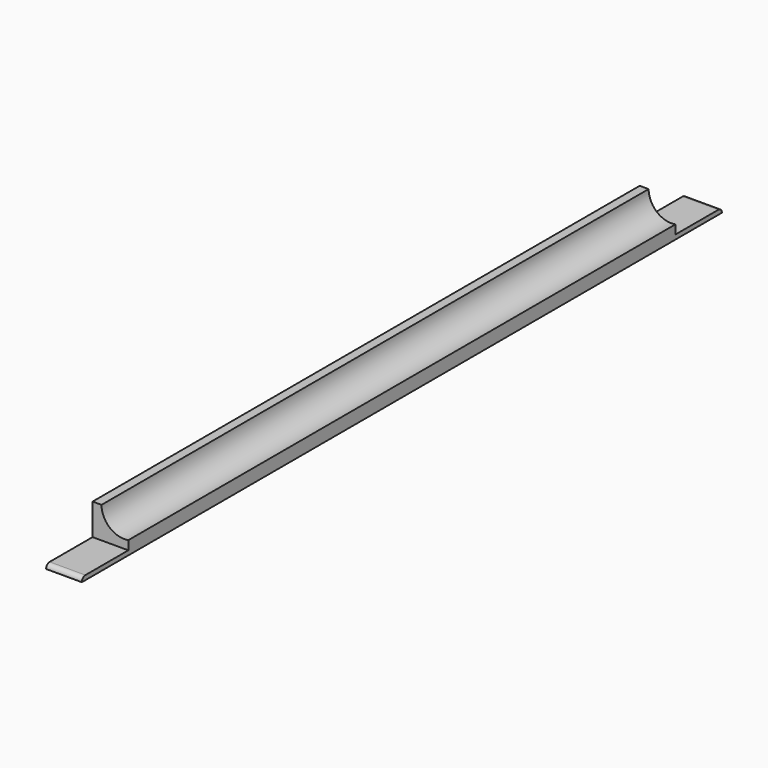
from build123d import *

# Parameters (mm, degrees)
F0_W     = 8
F0_H     = 153
F1_DEPTH = 7
F3_DEPTH = 160
F4_W     = 8
F4_H     = 179
F5_DEPTH = 1
F6_R     = 0.99999


# Not quite as in the source:
# - a fillet or chamfer is up to 0.001 mm smaller than in the source, because OpenCascade refuses the exact size


with BuildPart() as f1:
    # F0 (on Top) → F1 (new body)
    with BuildSketch(Plane.XY):
        Rectangle(F0_W, F0_H)
    extrude(amount=F1_DEPTH)

    # F2 (on face) → F3 (cut)
    with BuildSketch(Plane.XZ.offset(76.5)):
        with BuildLine():
            Line((4, 7), (-2, 7))
            ThreePointArc((-2, 7), (-0.1605232856, 3.1073720572), (4, 2))
            Line((4, 2), (4, 7))
        make_face()
    extrude(amount=-F3_DEPTH, mode=Mode.SUBTRACT)

    # F4 (on face) → F5 (join)
    with BuildSketch(Plane(origin=(0, 0, 0), x_dir=(1, 0, 0), z_dir=(0, 0, -1))):
        Rectangle(F4_W, F4_H)
    extrude(amount=F5_DEPTH)

    # F6 (radius 1 in the source; OpenCascade refuses exactly that, so slightly less here)
    f6_edges = [f1.edges().sort_by_distance(p)[0] for p in [
        (0, -89.5, 0),
        (0, 89.5, 0),
    ]]
    fillet(f6_edges, radius=F6_R)


solid = f1.part
